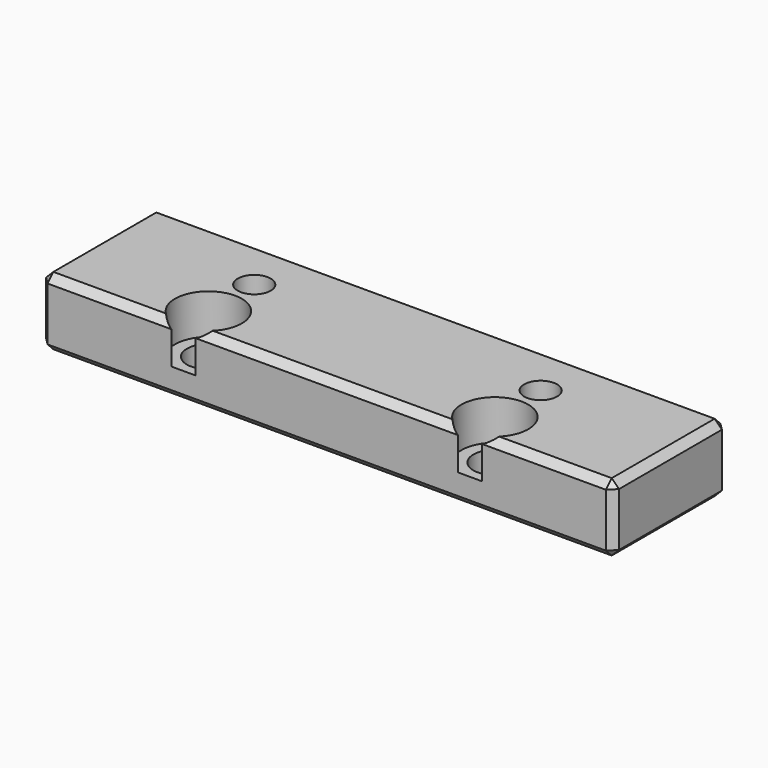
from build123d import *

# Parameters (mm, degrees)
F0_W           = 60
F0_H           = 15
F1_DEPTH       = 7.1374
F3_D           = 3.4544
F4_D           = 4.5
F4_CBORE_D     = 7
F4_CBORE_DEPTH = 4.2
F5_SIZE        = 0.762


with BuildPart() as f1:
    # F0 (on Top) → F1 (new body)
    with BuildSketch(Plane.XY):
        Rectangle(F0_W, F0_H)
    extrude(amount=F1_DEPTH)

    # F3 (through all)
    with Locations(Plane.XY.offset(7.1374)):
        with Locations((-15, 1.76), (15, 1.76)):
            Hole(F3_D / 2)

    # F4 (through all)
    with Locations(Plane.XY.offset(7.1374)):
        with Locations((-15, -4.24), (15, -4.24)):
            CounterBoreHole(F4_D / 2, F4_CBORE_D / 2, F4_CBORE_DEPTH)

    # F5
    f5_edges = [f1.edges().sort_by_distance(p)[0] for p in [
        (0, -7.5, 7.1374),
        (-30, 0, 7.1374),
        (0, 7.5, 7.1374),
        (30, 0, 7.1374),
        (30, -7.5, 3.5687),
        (30, 7.5, 3.5687),
        (30, 0, 0),
        (0, 7.5, 0),
        (-30, 7.5, 3.5687),
        (0, -7.5, 0),
        (-30, -7.5, 3.5687),
        (-30, 0, 0),
        (23.136867, -7.5, 7.1374),
        (-23.136867, -7.5, 7.1374),
    ]]
    chamfer(f5_edges, length=F5_SIZE)


solid = f1.part
